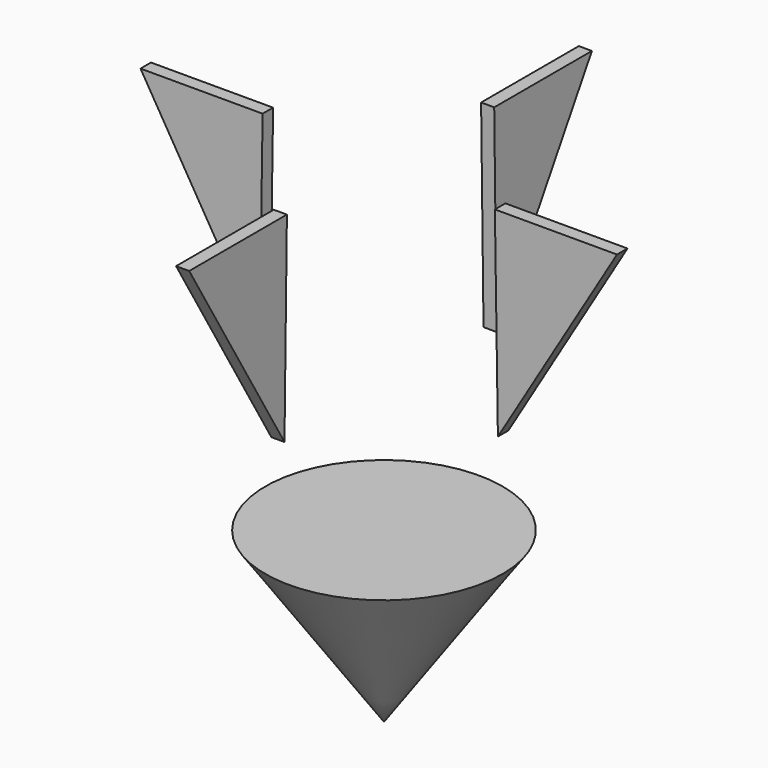
from build123d import *

# Parameters (mm, degrees)
F5_DEPTH = 2
F7_COUNT = 4


# Not quite as in the source:
# - the program builds the solid bodies; features that only make, move or delete a surface that nothing else refers to are left out


with BuildPart() as f3:
    # F2 (on Front) → F3 (revolve)
    with BuildSketch(Plane.XZ):
        Polygon((18.092494458, 0), (0, 0), (0, -25.7414802909), align=None)
    revolve(axis=Axis((0, 0, -12.8707401454), (0, 0, -1)))


with BuildPart() as f5:
    # F4 (on Right) → F5 (new body)
    with BuildSketch(Plane.YZ):
        Polygon((18.509125337, 49.8941615224), (18.9689788967, 19.5437967777), (37.1332131326, 49.8941615224), align=None)
    extrude(amount=F5_DEPTH)


with BuildPart() as f7_1:
    # F7: instance of F5
    add(f5.part.rotate(Axis((0, 0, 24.7171539813), (0, 0, 1)), 1 * 360 / F7_COUNT))


with BuildPart() as f7_2:
    # F7: instance of F5
    add(f5.part.rotate(Axis((0, 0, 24.7171539813), (0, 0, 1)), 2 * 360 / F7_COUNT))


with BuildPart() as f7_3:
    # F7: instance of F5
    add(f5.part.rotate(Axis((0, 0, 24.7171539813), (0, 0, 1)), 3 * 360 / F7_COUNT))


solid = Compound([f3.part, f5.part, f7_1.part, f7_2.part, f7_3.part])
